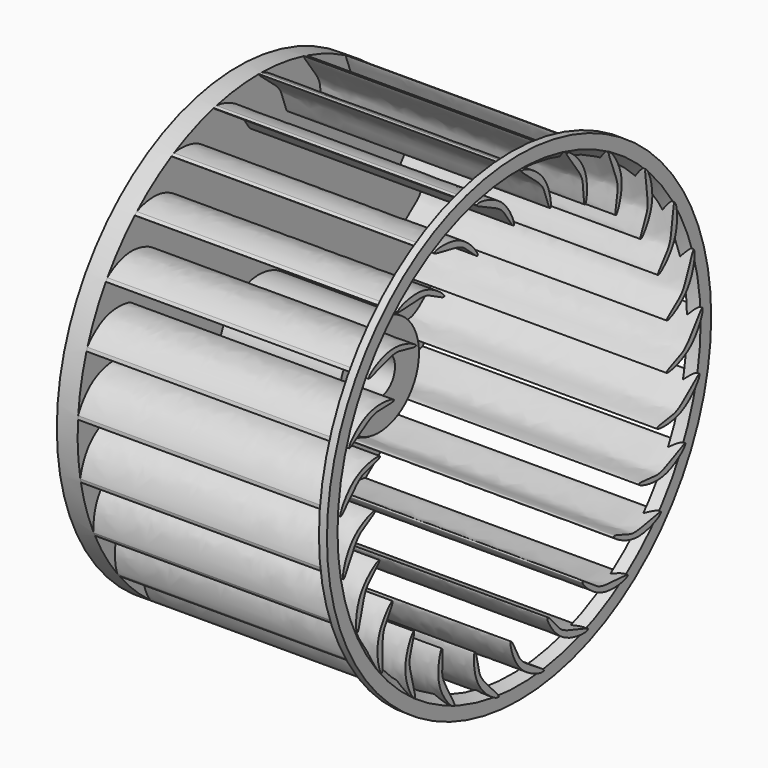
from build123d import *

# Parameters (mm, degrees)
F0_R            = 71.9026295482
F0_R_2          = 15.875
F1_DEPTH        = 12.7
F0_R_3          = 6.35
F2_DEPTH        = 50.8
F4_DEPTH        = 83.3162292838
F4_COPIES_COUNT = 25
F8_R            = 4.4227347534
F11_DEPTH       = 6.096


# Not quite as in the source:
# - a feature of the source that left no trace in its solid (it failed there, or was rolled back) is left out
# - a pattern or mirror of a feature is missing from the dataset's text; its kind, count and spacing are read off the source's solid


with BuildPart() as f1:
    # F0 (on Right) → F1 (new body)
    with BuildSketch(Plane.YZ):
        Circle(F0_R)
        Circle(F0_R_2, mode=Mode.SUBTRACT)
    extrude(amount=F1_DEPTH)

    # F0 (on Right) → F2 (join)
    with BuildSketch(Plane.YZ):
        Circle(F0_R_2)
        Circle(F0_R_3, mode=Mode.SUBTRACT)
    extrude(amount=F2_DEPTH)

    # F3 (on face) → F4 (join)
    with BuildSketch(Plane.YZ.offset(12.7)):
        with BuildLine():
            ThreePointArc((1.0952338885, 71.8942876638), (0.5476328281, 71.9005440469), (0, 71.9026295482))
            add(Edge.make_bspline(
                [(1.0952338885, 71.8942876638), (2.8691689683, 71.3621770641), (11.2039851865, 66.8319309701), (12.3591129927, 53.2113582075), (9.1768857575, 61.7596054259), (8.5785189706, 65.189757169), (-0.1118804815, 71.1858747547), (0, 71.9026295482)],
                knots=[0.061501835, 0.061501835, 0.061501835, 0.061501835, 0.229561248, 0.4595171174, 0.6113311303, 0.7753223155, 1, 1, 1, 1], degree=3))
        make_face()
    f4 = extrude(amount=F4_DEPTH)

    # F4_copies: F4 ×25 about axis
    f4_copies_axis = Axis((0, 0, 0), (1, 0, 0))
    for i in range(1, F4_COPIES_COUNT):
        add(f4.rotate(f4_copies_axis, i * 360 / F4_COPIES_COUNT))

    # F8 (on Top) → F9 (revolve, cut)
    with BuildSketch(Plane.XY):
        with Locations((-15.9850676343, 26.8231820053)):
            Circle(F8_R)
        Polygon((95.25, 76.2), (92.71, 76.2), (92.71, 69.85), (95.25, 72.009), align=None)
    revolve(axis=Axis((0, 0, 0), (-1, 0, 0)), mode=Mode.SUBTRACT)

    # F11 (cut): a face of the model
    f11_faces = [f1.faces().sort_by_distance(p)[0] for p in [
        (0, -69.8689160707, 0),
    ]]
    extrude(f11_faces, amount=-F11_DEPTH, mode=Mode.SUBTRACT)


with BuildPart() as f10:
    # F8 (on Top) → F10 (revolve)
    with BuildSketch(Plane.XY):
        Polygon((95.25, 76.2), (92.71, 76.2), (92.71, 69.85), (95.25, 72.009), align=None)
    revolve(axis=Axis((0, 0, 0), (-1, 0, 0)))


solid = Compound([f1.part, f10.part])
